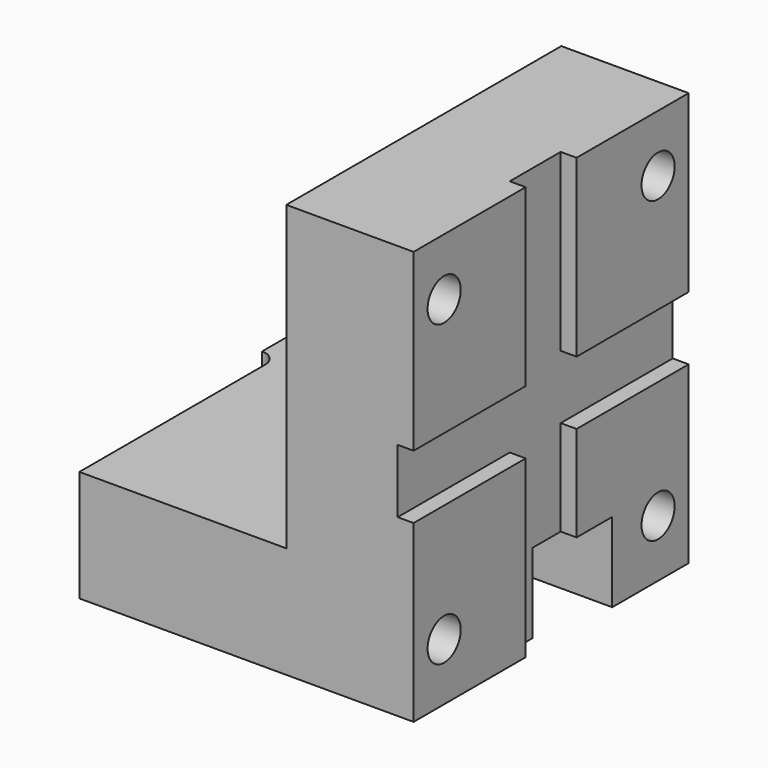
from build123d import *

# Parameters (mm, degrees)
F0_W      = 108
F0_H      = 130
F1_DEPTH  = 110
F2_R      = 6.5
F3_DEPTH  = 110.001
F4_W      = 108
F4_H      = 95
F5_DEPTH  = 70
F6_W      = 110
F6_H      = 25
F7_DEPTH  = 25
F8_R      = 6.5
F9_DEPTH  = 5
F10_R     = 4.99999
F11_R     = 10
F12_DEPTH = 20
F13_R     = 10
F14_DEPTH = 20
F15_W     = 20
F15_H     = 55
F15_W_2   = 44
F15_H_2   = 20
F16_DEPTH = 5


# Not quite as in the source:
# - a fillet or chamfer is up to 0.001 mm smaller than in the source, because OpenCascade refuses the exact size


with BuildPart() as f1:
    # F0 (on Right) → F1 (new body)
    with BuildSketch(Plane.YZ):
        Rectangle(F0_W, F0_H)
    extrude(amount=-F1_DEPTH)

    # F2 (on face) → F3 (cut, through all)
    with BuildSketch(Plane(origin=(-110, 0, 0), x_dir=(0, -1, 0), z_dir=(-1, 0, 0))):
        with Locations((-42, 47)):
            Circle(F2_R)
        with Locations((42, 47)):
            Circle(F2_R)
        with Locations((-42, -47)):
            Circle(F2_R)
        with Locations((42, -47)):
            Circle(F2_R)
    extrude(amount=-F3_DEPTH, mode=Mode.SUBTRACT)

    # F4 (on face) → F5 (cut)
    with BuildSketch(Plane(origin=(-110, 0, 0), x_dir=(0, -1, 0), z_dir=(-1, 0, 0))):
        with Locations((0, 17.5)):
            Rectangle(F4_W, F4_H)
    extrude(amount=-F5_DEPTH, mode=Mode.SUBTRACT)

    # F6 (on face) → F7 (cut)
    with BuildSketch(Plane(origin=(0, 0, -65), x_dir=(1, 0, 0), z_dir=(0, 0, -1))):
        with Locations((-55, -11.5)):
            Rectangle(F6_W, F6_H)
    extrude(amount=-F7_DEPTH, mode=Mode.SUBTRACT)

    # F8 (on face) → F9 (cut)
    with BuildSketch(Plane(origin=(-110, 0, 0), x_dir=(0, -1, 0), z_dir=(-1, 0, 0))):
        Polygon((-24, -30), (-24, -40), (1, -40), (1, -65), (54, -65), (54, -30), align=None)
        with Locations((42, -47)):
            Circle(F8_R, mode=Mode.SUBTRACT)
    extrude(amount=-F9_DEPTH, mode=Mode.SUBTRACT)

    # F10 (radius 5 in the source; OpenCascade refuses exactly that, so slightly less here)
    f10_edges = [f1.edges().sort_by_distance(p)[0] for p in [
        (-105, 24, -35),
    ]]
    fillet(f10_edges, radius=F10_R)

    # F11 (on face) → F12 (cut)
    with BuildSketch(Plane(origin=(-40, 0, 0), x_dir=(0, -1, 0), z_dir=(-1, 0, 0))):
        with Locations((-42, 47)):
            Circle(F11_R)
        with Locations((42, 47)):
            Circle(F11_R)
    extrude(amount=-F12_DEPTH, mode=Mode.SUBTRACT)

    # F13 (on face) → F14 (cut)
    with BuildSketch(Plane(origin=(-110, 0, 0), x_dir=(0, -1, 0), z_dir=(-1, 0, 0))):
        with Locations((-42, -47)):
            Circle(F13_R)
        with Locations((42, -47)):
            Circle(F13_R)
    extrude(amount=-F14_DEPTH, mode=Mode.SUBTRACT)

    # F15 (on face) → F16 (cut)
    with BuildSketch(Plane.YZ):
        with Locations((0, 37.5)):
            Rectangle(F15_W, F15_H)
        with Locations((32, 0)):
            Rectangle(F15_W_2, F15_H_2)
        Rectangle(F15_W, F15_H_2)
        with Locations((-32, 0)):
            Rectangle(F15_W_2, F15_H_2)
        with Locations((0, -37.5)):
            Rectangle(F15_W, F15_H)
    extrude(amount=-F16_DEPTH, mode=Mode.SUBTRACT)


solid = f1.part
